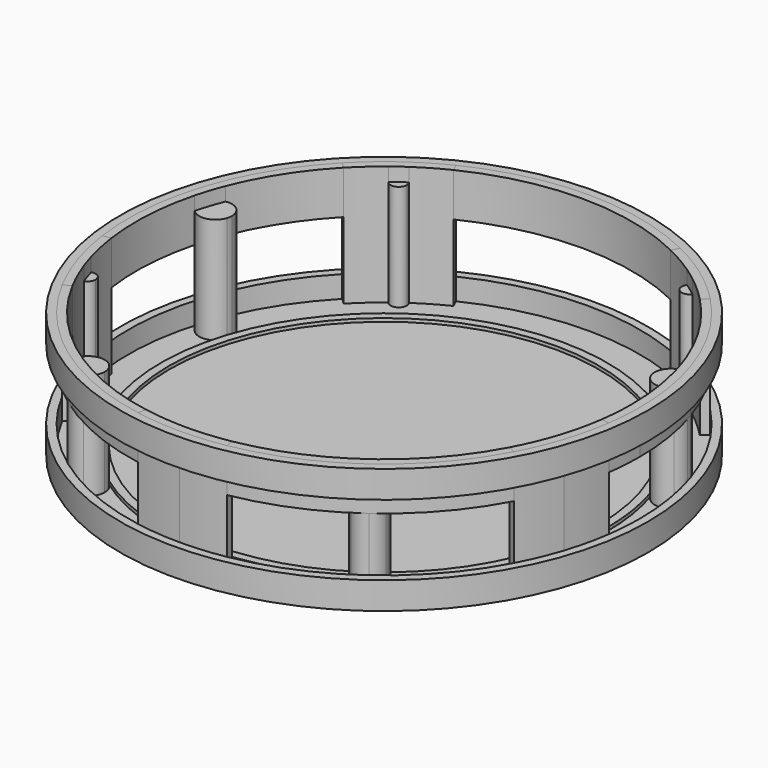
from build123d import *

# Parameters (mm, degrees)
F0_R     = 39.5
F1_DEPTH = 1
F2_DEPTH = 1.6
F3_DEPTH = 20.5
F4_DEPTH = 23
F5_START = 15
F5_DEPTH = 8
F0_R_2   = 48.5
F6_DEPTH = 5
F7_START = 18
F7_DEPTH = 5


with BuildPart() as f1:
    # F0 (on Top) → F1 (new body)
    with BuildSketch(Plane.XY):
        Circle(F0_R)
    extrude(amount=F1_DEPTH)


with BuildPart() as f1b:
    # F0 (on Top) → F1, piece 2 (new body)
    with BuildSketch(Plane.XY):
        with BuildLine():
            ThreePointArc((24.0991953374, -33.1696967742), (-9.68e-08, -41), (-24.099195494, -33.1696966604))
            ThreePointArc((-24.099195494, -33.1696966604), (-23.1895315704, -34.2347761707), (-22.8625511009, -35.5967477525))
            ThreePointArc((-22.8625511009, -35.5967477525), (-23.3228890862, -37.1936562819), (-24.5626290017, -38.3004863745))
            ThreePointArc((-24.5626290017, -38.3004863745), (-16.5547895287, -42.3814693429), (-7.9009920838, -44.8087527621))
            ThreePointArc((-7.9009920838, -44.8087527621), (-4.7121935446, -45.2553337409), (-1.4997962064, -45.4752747253))
            ThreePointArc((-1.4997962064, -45.4752747253), (0, -44), (1.4997962064, -45.4752747253))
            ThreePointArc((1.4997962064, -45.4752747253), (4.7121935446, -45.2553337409), (7.9009920838, -44.8087527621))
            ThreePointArc((7.9009920838, -44.8087527621), (16.5547895287, -42.3814693429), (24.5626290017, -38.3004863745))
            ThreePointArc((24.5626290017, -38.3004863745), (22.8747143756, -35.8666212476), (24.0991953374, -33.1696967742))
        make_face()
        with BuildLine():
            ThreePointArc((-24.5626290017, -38.3004863745), (-26.1324246507, -38.5845844728), (-27.6259069533, -38.0237986662))
            ThreePointArc((-27.6259069533, -38.0237986662), (-18.3643630933, -43.2637280892), (-8.1614643503, -46.2859643916))
            Line((-8.1614643503, -46.2859643916), (-7.9009920838, -44.8087527621))
            ThreePointArc((-7.9009920838, -44.8087527621), (-16.5547895287, -42.3814693429), (-24.5626290017, -38.3004863745))
        make_face()
        with BuildLine():
            ThreePointArc((8.1614643503, -46.2859643916), (18.3643629027, -43.2637281701), (27.6259066181, -38.0237989097))
            ThreePointArc((27.6259066181, -38.0237989097), (26.1324244444, -38.5845844914), (24.5626290017, -38.3004863745))
            ThreePointArc((24.5626290017, -38.3004863745), (16.5547895287, -42.3814693429), (7.9009920838, -44.8087527621))
            Line((7.9009920838, -44.8087527621), (8.1614643503, -46.2859643916))
        make_face()
    extrude(amount=F1_DEPTH)


with BuildPart() as f1c:
    # F0 (on Top) → F1, piece 3 (new body)
    with BuildSketch(Plane.XY):
        with BuildLine():
            ThreePointArc((45.5, 0), (45.1275246407, 5.8100361274), (44.0161969318, 11.5249471869))
            ThreePointArc((44.0161969318, 11.5249471869), (41.1798592989, 10.6717506781), (38.9933171455, 12.669696839))
            ThreePointArc((38.9933171455, 12.669696839), (40.4952219587, 6.4138131028), (41, 0))
            ThreePointArc((41, 0), (36.5312674899, -18.613610493), (24.0991953374, -33.1696967742))
            ThreePointArc((24.0991953374, -33.1696967742), (27.0425083639, -32.8385416584), (28.8356573557, -35.195949552))
            ThreePointArc((28.8356573557, -35.195949552), (35.191461286, -28.8411347307), (40.1741154751, -21.3609561068))
            ThreePointArc((40.1741154751, -21.3609561068), (41.5842321653, -18.4662295886), (42.7860938419, -15.4790236692))
            ThreePointArc((42.7860938419, -15.4790236692), (41.846486717, -13.5967477525), (43.7130188737, -12.6262417587))
            ThreePointArc((43.7130188737, -12.6262417587), (44.4965279374, -9.5031048354), (45.0571971277, -6.3323760937))
            ThreePointArc((45.0571971277, -6.3323760937), (45.3891642868, -3.1739195554), (45.5, 0))
        make_face()
        with BuildLine():
            ThreePointArc((27.6259066181, -38.0237989097), (35.4713501733, -30.8347744743), (41.4985368644, -22.0651634509))
            Line((41.4985368644, -22.0651634509), (40.1741154751, -21.3609561068))
            ThreePointArc((40.1741154751, -21.3609561068), (35.191461286, -28.8411347307), (28.8356573557, -35.195949552))
            ThreePointArc((28.8356573557, -35.195949552), (28.8558201135, -35.3958980132), (28.8625511009, -35.5967477525))
            ThreePointArc((28.8625511009, -35.5967477525), (28.5355706062, -36.9587193837), (27.6259066181, -38.0237989097))
        make_face()
        with BuildLine():
            ThreePointArc((47, 0), (46.4213520001, 7.3524199067), (44.6996562347, 14.5237988315))
            ThreePointArc((44.6996562347, 14.5237988315), (44.8095517309, 14.0660511974), (44.846486717, 13.5967477525))
            ThreePointArc((44.846486717, 13.5967477525), (44.6311887338, 12.4807573055), (44.0161969318, 11.5249471869))
            ThreePointArc((44.0161969318, 11.5249471869), (45.1275246407, 5.8100361274), (45.5, 0))
            ThreePointArc((45.5, 0), (45.3891642868, -3.1739195554), (45.0571971277, -6.3323760937))
            Line((45.0571971277, -6.3323760937), (46.5425992309, -6.5411357451))
            ThreePointArc((46.5425992309, -6.5411357451), (46.8855103622, -3.278554266), (47, 0))
        make_face()
    extrude(amount=F1_DEPTH)


with BuildPart() as f1d:
    # F0 (on Top) → F1, piece 4 (new body)
    with BuildSketch(Plane.XY):
        with BuildLine():
            ThreePointArc((25.5163352084, 37.6718281682), (22.7881731021, 39.3820919539), (19.9458871789, 40.8951291066))
            ThreePointArc((19.9458871789, 40.8951291066), (0, 45.5), (-19.9458871789, 40.8951291066))
            ThreePointArc((-19.9458871789, 40.8951291066), (-22.7881731021, 39.3820919539), (-25.5163352084, 37.6718281682))
            ThreePointArc((-25.5163352084, 37.6718281682), (-25.3138722657, 37.2620250252), (-25.2442289793, 36.8102732441))
            ThreePointArc((-25.2442289793, 36.8102732441), (-26.2689612657, 35.38755732), (-27.9430564466, 35.908711985))
            ThreePointArc((-27.9430564466, 35.908711985), (-30.4126624188, 33.842576211), (-32.7299609154, 31.6069558559))
            ThreePointArc((-32.7299609154, 31.6069558559), (-38.3043087172, 24.5566678052), (-42.3840453355, 16.5481932851))
            ThreePointArc((-42.3840453355, 16.5481932851), (-39.9245964828, 15.9002967378), (-38.846486717, 13.5967477525))
            ThreePointArc((-38.846486717, 13.5967477525), (-38.8834216837, 13.12744443), (-38.9933171226, 12.6696969093))
            ThreePointArc((-38.9933171226, 12.6696969093), (3.7e-08, 41), (38.9933171455, 12.669696839))
            ThreePointArc((38.9933171455, 12.669696839), (39.5879037117, 15.5712863842), (42.3840453355, 16.5481932851))
            ThreePointArc((42.3840453355, 16.5481932851), (38.3043087172, 24.5566678052), (32.7299609154, 31.6069558559))
            ThreePointArc((32.7299609154, 31.6069558559), (30.4126624188, 33.842576211), (27.9430564466, 35.908711985))
            ThreePointArc((27.9430564466, 35.908711985), (25.8625511009, 35.5967477525), (25.5163352084, 37.6718281682))
        make_face()
        with BuildLine():
            ThreePointArc((44.6996562347, 14.5237988315), (40.286863107, 24.206789564), (33.8089706159, 32.6489434116))
            Line((33.8089706159, 32.6489434116), (32.7299609154, 31.6069558559))
            ThreePointArc((32.7299609154, 31.6069558559), (38.3043087172, 24.5566678052), (42.3840453355, 16.5481932851))
            ThreePointArc((42.3840453355, 16.5481932851), (43.8210252832, 15.8553308151), (44.6996562347, 14.5237988315))
        make_face()
        with BuildLine():
            Line((19.9458871789, 40.8951291066), (20.6034438991, 42.2433201761))
            ThreePointArc((20.6034438991, 42.2433201761), (0, 47), (-20.6034438991, 42.2433201761))
            Line((-20.6034438991, 42.2433201761), (-19.9458871789, 40.8951291066))
            ThreePointArc((-19.9458871789, 40.8951291066), (0, 45.5), (19.9458871789, 40.8951291066))
        make_face()
        with BuildLine():
            Line((-32.7299609154, 31.6069558559), (-33.8089706159, 32.6489434116))
            ThreePointArc((-33.8089706159, 32.6489434116), (-40.2868630773, 24.2067896134), (-44.6996561991, 14.5237989412))
            ThreePointArc((-44.6996561991, 14.5237989412), (-43.8210252397, 15.8553308531), (-42.3840453355, 16.5481932851))
            ThreePointArc((-42.3840453355, 16.5481932851), (-38.3043087172, 24.5566678052), (-32.7299609154, 31.6069558559))
        make_face()
    extrude(amount=F1_DEPTH)


with BuildPart() as f1e:
    # F0 (on Top) → F1, piece 5 (new body)
    with BuildSketch(Plane.XY):
        with BuildLine():
            ThreePointArc((-38.9933171226, 12.6696969093), (-41.1798592628, 10.6717506863), (-44.0161969318, 11.5249471869))
            ThreePointArc((-44.0161969318, 11.5249471869), (-45.4228838914, 2.6479461836), (-45.0571971277, -6.3323760937))
            ThreePointArc((-45.0571971277, -6.3323760937), (-44.4965279374, -9.5031048354), (-43.7130188737, -12.6262417587))
            ThreePointArc((-43.7130188737, -12.6262417587), (-42.3814216368, -12.8540557941), (-41.7730714914, -14.0602732441))
            ThreePointArc((-41.7730714914, -14.0602732441), (-42.0523203959, -14.9319192518), (-42.7860938419, -15.4790236692))
            ThreePointArc((-42.7860938419, -15.4790236692), (-41.5842321653, -18.4662295886), (-40.1741154751, -21.3609561068))
            ThreePointArc((-40.1741154751, -21.3609561068), (-35.191461286, -28.8411347307), (-28.8356573557, -35.195949552))
            ThreePointArc((-28.8356573557, -35.195949552), (-27.0425084529, -32.8385416965), (-24.099195494, -33.1696966604))
            ThreePointArc((-24.099195494, -33.1696966604), (-38.9933172195, -12.6696966113), (-38.9933171226, 12.6696969093))
        make_face()
        with BuildLine():
            Line((-40.1741154751, -21.3609561068), (-41.4985368644, -22.0651634509))
            ThreePointArc((-41.4985368644, -22.0651634509), (-35.4713503092, -30.834774318), (-27.6259069533, -38.0237986662))
            ThreePointArc((-27.6259069533, -38.0237986662), (-28.6207572165, -36.7767049651), (-28.8356573557, -35.195949552))
            ThreePointArc((-28.8356573557, -35.195949552), (-35.191461286, -28.8411347307), (-40.1741154751, -21.3609561068))
        make_face()
        with BuildLine():
            ThreePointArc((-44.0161969318, 11.5249471869), (-44.7714838236, 12.9301204755), (-44.6996561991, 14.5237989412))
            ThreePointArc((-44.6996561991, 14.5237989412), (-46.8211508009, 4.0963200168), (-46.5425992309, -6.5411357451))
            Line((-46.5425992309, -6.5411357451), (-45.0571971277, -6.3323760937))
            ThreePointArc((-45.0571971277, -6.3323760937), (-45.4228838914, 2.6479461836), (-44.0161969318, 11.5249471869))
        make_face()
    extrude(amount=F1_DEPTH)


with BuildPart() as f2:
    # F0 (on Top) → F2 (new body)
    with BuildSketch(Plane.XY):
        with BuildLine():
            ThreePointArc((41, 0), (40.4952219587, 6.4138131028), (38.9933171455, 12.669696839))
            ThreePointArc((38.9933171455, 12.669696839), (3.7e-08, 41), (-38.9933171226, 12.6696969093))
            ThreePointArc((-38.9933171226, 12.6696969093), (-38.9933172195, -12.6696966113), (-24.099195494, -33.1696966604))
            ThreePointArc((-24.099195494, -33.1696966604), (-9.68e-08, -41), (24.0991953374, -33.1696967742))
            ThreePointArc((24.0991953374, -33.1696967742), (36.5312674899, -18.613610493), (41, 0))
        make_face()
        Circle(F0_R, mode=Mode.SUBTRACT)
    extrude(amount=F2_DEPTH)


with BuildPart() as f3:
    # F0 (on Top) → F3 (new body)
    with BuildSketch(Plane.XY):
        with BuildLine():
            ThreePointArc((27.9430564466, 35.908711985), (26.7442289793, 36.8102732441), (25.5163352084, 37.6718281682))
            ThreePointArc((25.5163352084, 37.6718281682), (25.8625511009, 35.5967477525), (27.9430564466, 35.908711985))
        make_face()
    extrude(amount=F3_DEPTH)


with BuildPart() as f3b:
    # F0 (on Top) → F3, piece 2 (new body)
    with BuildSketch(Plane.XY):
        with BuildLine():
            ThreePointArc((-25.2442289793, 36.8102732441), (-25.3138722657, 37.2620250252), (-25.5163352084, 37.6718281682))
            ThreePointArc((-25.5163352084, 37.6718281682), (-26.7442289793, 36.8102732441), (-27.9430564466, 35.908711985))
            ThreePointArc((-27.9430564466, 35.908711985), (-26.2689612657, 35.38755732), (-25.2442289793, 36.8102732441))
        make_face()
    extrude(amount=F3_DEPTH)


with BuildPart() as f3c:
    # F0 (on Top) → F3, piece 3 (new body)
    with BuildSketch(Plane.XY):
        with BuildLine():
            ThreePointArc((44.846486717, 13.5967477525), (44.8095517309, 14.0660511974), (44.6996562347, 14.5237988315))
            ThreePointArc((44.6996562347, 14.5237988315), (43.8210252832, 15.8553308151), (42.3840453355, 16.5481932851))
            ThreePointArc((42.3840453355, 16.5481932851), (43.2730714914, 14.0602732441), (44.0161969318, 11.5249471869))
            ThreePointArc((44.0161969318, 11.5249471869), (44.6311887338, 12.4807573055), (44.846486717, 13.5967477525))
        make_face()
        with BuildLine():
            ThreePointArc((44.0161969318, 11.5249471869), (43.2730714914, 14.0602732441), (42.3840453355, 16.5481932851))
            ThreePointArc((42.3840453355, 16.5481932851), (39.5879037117, 15.5712863842), (38.9933171455, 12.669696839))
            ThreePointArc((38.9933171455, 12.669696839), (41.1798592989, 10.6717506781), (44.0161969318, 11.5249471869))
        make_face()
    extrude(amount=F3_DEPTH)


with BuildPart() as f3d:
    # F0 (on Top) → F3, piece 4 (new body)
    with BuildSketch(Plane.XY):
        with BuildLine():
            ThreePointArc((-42.3840453355, 16.5481932851), (-43.8210252397, 15.8553308531), (-44.6996561991, 14.5237989412))
            ThreePointArc((-44.6996561991, 14.5237989412), (-44.7714838236, 12.9301204755), (-44.0161969318, 11.5249471869))
            ThreePointArc((-44.0161969318, 11.5249471869), (-43.2730714914, 14.0602732441), (-42.3840453355, 16.5481932851))
        make_face()
        with BuildLine():
            ThreePointArc((-38.846486717, 13.5967477525), (-39.9245964828, 15.9002967378), (-42.3840453355, 16.5481932851))
            ThreePointArc((-42.3840453355, 16.5481932851), (-43.2730714914, 14.0602732441), (-44.0161969318, 11.5249471869))
            ThreePointArc((-44.0161969318, 11.5249471869), (-41.1798592628, 10.6717506863), (-38.9933171226, 12.6696969093))
            ThreePointArc((-38.9933171226, 12.6696969093), (-38.8834216837, 13.12744443), (-38.846486717, 13.5967477525))
        make_face()
    extrude(amount=F3_DEPTH)


with BuildPart() as f3e:
    # F0 (on Top) → F3, piece 5 (new body)
    with BuildSketch(Plane.XY):
        with BuildLine():
            ThreePointArc((-41.7730714914, -14.0602732441), (-42.3814216368, -12.8540557941), (-43.7130188737, -12.6262417587))
            ThreePointArc((-43.7130188737, -12.6262417587), (-43.2730714914, -14.0602732441), (-42.7860938419, -15.4790236692))
            ThreePointArc((-42.7860938419, -15.4790236692), (-42.0523203959, -14.9319192518), (-41.7730714914, -14.0602732441))
        make_face()
    extrude(amount=F3_DEPTH)


with BuildPart() as f3f:
    # F0 (on Top) → F3, piece 6 (new body)
    with BuildSketch(Plane.XY):
        with BuildLine():
            ThreePointArc((-22.8625511009, -35.5967477525), (-23.1895315704, -34.2347761707), (-24.099195494, -33.1696966604))
            ThreePointArc((-24.099195494, -33.1696966604), (-27.0425084529, -32.8385416965), (-28.8356573557, -35.195949552))
            ThreePointArc((-28.8356573557, -35.195949552), (-26.7442289793, -36.8102732441), (-24.5626290017, -38.3004863745))
            ThreePointArc((-24.5626290017, -38.3004863745), (-23.3228890862, -37.1936562819), (-22.8625511009, -35.5967477525))
        make_face()
        with BuildLine():
            ThreePointArc((-28.8356573557, -35.195949552), (-28.6207572165, -36.7767049651), (-27.6259069533, -38.0237986662))
            ThreePointArc((-27.6259069533, -38.0237986662), (-26.1324246507, -38.5845844728), (-24.5626290017, -38.3004863745))
            ThreePointArc((-24.5626290017, -38.3004863745), (-26.7442289793, -36.8102732441), (-28.8356573557, -35.195949552))
        make_face()
    extrude(amount=F3_DEPTH)


with BuildPart() as f3g:
    # F0 (on Top) → F3, piece 7 (new body)
    with BuildSketch(Plane.XY):
        with BuildLine():
            ThreePointArc((43.7130188737, -12.6262417587), (41.846486717, -13.5967477525), (42.7860938419, -15.4790236692))
            ThreePointArc((42.7860938419, -15.4790236692), (43.2730714914, -14.0602732441), (43.7130188737, -12.6262417587))
        make_face()
    extrude(amount=F3_DEPTH)


with BuildPart() as f3h:
    # F0 (on Top) → F3, piece 8 (new body)
    with BuildSketch(Plane.XY):
        with BuildLine():
            ThreePointArc((28.8356573557, -35.195949552), (27.0425083639, -32.8385416584), (24.0991953374, -33.1696967742))
            ThreePointArc((24.0991953374, -33.1696967742), (22.8747143756, -35.8666212476), (24.5626290017, -38.3004863745))
            ThreePointArc((24.5626290017, -38.3004863745), (26.7442289793, -36.8102732441), (28.8356573557, -35.195949552))
        make_face()
        with BuildLine():
            ThreePointArc((24.5626290017, -38.3004863745), (26.1324244444, -38.5845844914), (27.6259066181, -38.0237989097))
            ThreePointArc((27.6259066181, -38.0237989097), (28.5355706062, -36.9587193837), (28.8625511009, -35.5967477525))
            ThreePointArc((28.8625511009, -35.5967477525), (28.8558201135, -35.3958980132), (28.8356573557, -35.195949552))
            ThreePointArc((28.8356573557, -35.195949552), (26.7442289793, -36.8102732441), (24.5626290017, -38.3004863745))
        make_face()
    extrude(amount=F3_DEPTH)


with BuildPart() as f3i:
    # F0 (on Top) → F3, piece 9 (new body)
    with BuildSketch(Plane.XY):
        with BuildLine():
            ThreePointArc((0, -45.5), (0.75, -45.4938182614), (1.4997962064, -45.4752747253))
            ThreePointArc((1.4997962064, -45.4752747253), (0, -44), (-1.4997962064, -45.4752747253))
            ThreePointArc((-1.4997962064, -45.4752747253), (-0.75, -45.4938182614), (0, -45.5))
        make_face()
    extrude(amount=F3_DEPTH)


with BuildPart() as f4:
    # F0 (on Top) → F4 (new body)
    with BuildSketch(Plane.XY):
        with BuildLine():
            ThreePointArc((-42.7860938419, -15.4790236692), (-43.9430185539, -15.4023503408), (-44.6996562714, -14.5237987185))
            ThreePointArc((-44.6996562714, -14.5237987185), (-43.2637281158, -18.3643630307), (-41.4985368644, -22.0651634509))
            Line((-41.4985368644, -22.0651634509), (-40.1741154751, -21.3609561068))
            ThreePointArc((-40.1741154751, -21.3609561068), (-41.5842321653, -18.4662295886), (-42.7860938419, -15.4790236692))
        make_face()
        with BuildLine():
            ThreePointArc((-43.7130188737, -12.6262417587), (-44.6039231669, -13.3682950523), (-44.6996562714, -14.5237987185))
            ThreePointArc((-44.6996562714, -14.5237987185), (-43.9430185539, -15.4023503408), (-42.7860938419, -15.4790236692))
            ThreePointArc((-42.7860938419, -15.4790236692), (-43.2730714914, -14.0602732441), (-43.7130188737, -12.6262417587))
        make_face()
        with BuildLine():
            Line((-45.0571971277, -6.3323760937), (-46.5425992309, -6.5411357451))
            ThreePointArc((-46.5425992309, -6.5411357451), (-45.7953930469, -10.5726995454), (-44.6996562714, -14.5237987185))
            ThreePointArc((-44.6996562714, -14.5237987185), (-44.6039231669, -13.3682950523), (-43.7130188737, -12.6262417587))
            ThreePointArc((-43.7130188737, -12.6262417587), (-44.4965279374, -9.5031048354), (-45.0571971277, -6.3323760937))
        make_face()
    extrude(amount=F4_DEPTH)


with BuildPart() as f4b:
    # F0 (on Top) → F4, piece 2 (new body)
    with BuildSketch(Plane.XY):
        with BuildLine():
            ThreePointArc((-27.9430564466, 35.908711985), (-28.2276451659, 37.0327061945), (-27.6259067422, 38.0237988196))
            ThreePointArc((-27.6259067422, 38.0237988196), (-30.8347743086, 35.4713503173), (-33.8089706159, 32.6489434116))
            Line((-33.8089706159, 32.6489434116), (-32.7299609154, 31.6069558559))
            ThreePointArc((-32.7299609154, 31.6069558559), (-30.4126624188, 33.842576211), (-27.9430564466, 35.908711985))
        make_face()
        with BuildLine():
            ThreePointArc((-25.5163352084, 37.6718281682), (-26.497374334, 38.289821413), (-27.6259067422, 38.0237988196))
            ThreePointArc((-27.6259067422, 38.0237988196), (-28.2276451659, 37.0327061945), (-27.9430564466, 35.908711985))
            ThreePointArc((-27.9430564466, 35.908711985), (-26.7442289793, 36.8102732441), (-25.5163352084, 37.6718281682))
        make_face()
        with BuildLine():
            Line((-19.9458871789, 40.8951291066), (-20.6034438991, 42.2433201761))
            ThreePointArc((-20.6034438991, 42.2433201761), (-24.2067894595, 40.2868631698), (-27.6259067422, 38.0237988196))
            ThreePointArc((-27.6259067422, 38.0237988196), (-26.497374334, 38.289821413), (-25.5163352084, 37.6718281682))
            ThreePointArc((-25.5163352084, 37.6718281682), (-22.7881731021, 39.3820919539), (-19.9458871789, 40.8951291066))
        make_face()
    extrude(amount=F4_DEPTH)


with BuildPart() as f4c:
    # F0 (on Top) → F4, piece 3 (new body)
    with BuildSketch(Plane.XY):
        with BuildLine():
            ThreePointArc((28.2442289793, 36.8102732441), (28.0807387591, 37.4912590064), (27.6259068347, 38.0237987524))
            ThreePointArc((27.6259068347, 38.0237987524), (26.4973743904, 38.2898214224), (25.5163352084, 37.6718281682))
            ThreePointArc((25.5163352084, 37.6718281682), (26.7442289793, 36.8102732441), (27.9430564466, 35.908711985))
            ThreePointArc((27.9430564466, 35.908711985), (28.1669449033, 36.3350055305), (28.2442289793, 36.8102732441))
        make_face()
        with BuildLine():
            ThreePointArc((27.6259068347, 38.0237987524), (24.2067895086, 40.2868631403), (20.6034438991, 42.2433201761))
            Line((20.6034438991, 42.2433201761), (19.9458871789, 40.8951291066))
            ThreePointArc((19.9458871789, 40.8951291066), (22.7881731021, 39.3820919539), (25.5163352084, 37.6718281682))
            ThreePointArc((25.5163352084, 37.6718281682), (26.4973743904, 38.2898214224), (27.6259068347, 38.0237987524))
        make_face()
        with BuildLine():
            ThreePointArc((33.8089706159, 32.6489434116), (30.8347743518, 35.4713502798), (27.6259068347, 38.0237987524))
            ThreePointArc((27.6259068347, 38.0237987524), (28.0807387591, 37.4912590064), (28.2442289793, 36.8102732441))
            ThreePointArc((28.2442289793, 36.8102732441), (28.1669449033, 36.3350055305), (27.9430564466, 35.908711985))
            ThreePointArc((27.9430564466, 35.908711985), (30.4126624188, 33.842576211), (32.7299609154, 31.6069558559))
            Line((32.7299609154, 31.6069558559), (33.8089706159, 32.6489434116))
        make_face()
    extrude(amount=F4_DEPTH)


with BuildPart() as f4d:
    # F0 (on Top) → F4, piece 4 (new body)
    with BuildSketch(Plane.XY):
        with BuildLine():
            ThreePointArc((42.7860938419, -15.4790236692), (43.9430184652, -15.402350385), (44.6996562102, -14.523798907))
            ThreePointArc((44.6996562102, -14.523798907), (44.7546039882, -14.2949250306), (44.7730714914, -14.0602732441))
            ThreePointArc((44.7730714914, -14.0602732441), (44.4792889414, -13.1686233894), (43.7130188737, -12.6262417587))
            ThreePointArc((43.7130188737, -12.6262417587), (43.2730714914, -14.0602732441), (42.7860938419, -15.4790236692))
        make_face()
        with BuildLine():
            ThreePointArc((44.6996562102, -14.523798907), (45.7953930246, -10.572699642), (46.5425992309, -6.5411357451))
            Line((46.5425992309, -6.5411357451), (45.0571971277, -6.3323760937))
            ThreePointArc((45.0571971277, -6.3323760937), (44.4965279374, -9.5031048354), (43.7130188737, -12.6262417587))
            ThreePointArc((43.7130188737, -12.6262417587), (44.4792889414, -13.1686233894), (44.7730714914, -14.0602732441))
            ThreePointArc((44.7730714914, -14.0602732441), (44.7546039882, -14.2949250306), (44.6996562102, -14.523798907))
        make_face()
        with BuildLine():
            ThreePointArc((41.4985368644, -22.0651634509), (43.2637280771, -18.3643631219), (44.6996562102, -14.523798907))
            ThreePointArc((44.6996562102, -14.523798907), (43.9430184652, -15.402350385), (42.7860938419, -15.4790236692))
            ThreePointArc((42.7860938419, -15.4790236692), (41.5842321653, -18.4662295886), (40.1741154751, -21.3609561068))
            Line((40.1741154751, -21.3609561068), (41.4985368644, -22.0651634509))
        make_face()
    extrude(amount=F4_DEPTH)


with BuildPart() as f4e:
    # F0 (on Top) → F4, piece 5 (new body)
    with BuildSketch(Plane.XY):
        with BuildLine():
            ThreePointArc((-1.4997962064, -45.4752747253), (-1.0693661469, -46.5518821436), (0, -47))
            Line((0, -47), (0, -45.5))
            ThreePointArc((0, -45.5), (-0.75, -45.4938182614), (-1.4997962064, -45.4752747253))
        make_face()
        with BuildLine():
            Line((0, -45.5), (0, -47))
            ThreePointArc((0, -47), (1.0606601718, -46.5606601718), (1.5, -45.5))
            ThreePointArc((1.5, -45.5), (1.4999490507, -45.4876369427), (1.4997962064, -45.4752747253))
            ThreePointArc((1.4997962064, -45.4752747253), (0.75, -45.4938182614), (0, -45.5))
        make_face()
        with BuildLine():
            ThreePointArc((0, -47), (4.0963199091, -46.8211508103), (8.1614643503, -46.2859643916))
            Line((8.1614643503, -46.2859643916), (7.9009920838, -44.8087527621))
            ThreePointArc((7.9009920838, -44.8087527621), (4.7121935446, -45.2553337409), (1.4997962064, -45.4752747253))
            ThreePointArc((1.4997962064, -45.4752747253), (1.4999490507, -45.4876369427), (1.5, -45.5))
            ThreePointArc((1.5, -45.5), (1.0606601718, -46.5606601718), (0, -47))
        make_face()
        with BuildLine():
            Line((-7.9009920838, -44.8087527621), (-8.1614643503, -46.2859643916))
            ThreePointArc((-8.1614643503, -46.2859643916), (-4.0963199091, -46.8211508103), (0, -47))
            ThreePointArc((0, -47), (-1.0693661469, -46.5518821436), (-1.4997962064, -45.4752747253))
            ThreePointArc((-1.4997962064, -45.4752747253), (-4.7121935446, -45.2553337409), (-7.9009920838, -44.8087527621))
        make_face()
    extrude(amount=F4_DEPTH)


with BuildPart() as f5:
    # F0 (on Top) → F5 (new body)
    with BuildSketch(Plane.XY.offset(F5_START)):
        with BuildLine():
            ThreePointArc((-42.3840453355, 16.5481932851), (-43.8210252397, 15.8553308531), (-44.6996561991, 14.5237989412))
            ThreePointArc((-44.6996561991, 14.5237989412), (-44.7714838236, 12.9301204755), (-44.0161969318, 11.5249471869))
            ThreePointArc((-44.0161969318, 11.5249471869), (-43.2730714914, 14.0602732441), (-42.3840453355, 16.5481932851))
        make_face()
        with BuildLine():
            Line((-32.7299609154, 31.6069558559), (-33.8089706159, 32.6489434116))
            ThreePointArc((-33.8089706159, 32.6489434116), (-40.2868630773, 24.2067896134), (-44.6996561991, 14.5237989412))
            ThreePointArc((-44.6996561991, 14.5237989412), (-43.8210252397, 15.8553308531), (-42.3840453355, 16.5481932851))
            ThreePointArc((-42.3840453355, 16.5481932851), (-38.3043087172, 24.5566678052), (-32.7299609154, 31.6069558559))
        make_face()
        with BuildLine():
            ThreePointArc((-44.0161969318, 11.5249471869), (-44.7714838236, 12.9301204755), (-44.6996561991, 14.5237989412))
            ThreePointArc((-44.6996561991, 14.5237989412), (-46.8211508009, 4.0963200168), (-46.5425992309, -6.5411357451))
            Line((-46.5425992309, -6.5411357451), (-45.0571971277, -6.3323760937))
            ThreePointArc((-45.0571971277, -6.3323760937), (-45.4228838914, 2.6479461836), (-44.0161969318, 11.5249471869))
        make_face()
    extrude(amount=F5_DEPTH)


with BuildPart() as f5b:
    # F0 (on Top) → F5, piece 2 (new body)
    with BuildSketch(Plane.XY.offset(F5_START)):
        with BuildLine():
            ThreePointArc((-28.8356573557, -35.195949552), (-28.6207572165, -36.7767049651), (-27.6259069533, -38.0237986662))
            ThreePointArc((-27.6259069533, -38.0237986662), (-26.1324246507, -38.5845844728), (-24.5626290017, -38.3004863745))
            ThreePointArc((-24.5626290017, -38.3004863745), (-26.7442289793, -36.8102732441), (-28.8356573557, -35.195949552))
        make_face()
        with BuildLine():
            Line((-40.1741154751, -21.3609561068), (-41.4985368644, -22.0651634509))
            ThreePointArc((-41.4985368644, -22.0651634509), (-35.4713503092, -30.834774318), (-27.6259069533, -38.0237986662))
            ThreePointArc((-27.6259069533, -38.0237986662), (-28.6207572165, -36.7767049651), (-28.8356573557, -35.195949552))
            ThreePointArc((-28.8356573557, -35.195949552), (-35.191461286, -28.8411347307), (-40.1741154751, -21.3609561068))
        make_face()
        with BuildLine():
            ThreePointArc((-24.5626290017, -38.3004863745), (-26.1324246507, -38.5845844728), (-27.6259069533, -38.0237986662))
            ThreePointArc((-27.6259069533, -38.0237986662), (-18.3643630933, -43.2637280892), (-8.1614643503, -46.2859643916))
            Line((-8.1614643503, -46.2859643916), (-7.9009920838, -44.8087527621))
            ThreePointArc((-7.9009920838, -44.8087527621), (-16.5547895287, -42.3814693429), (-24.5626290017, -38.3004863745))
        make_face()
    extrude(amount=F5_DEPTH)


with BuildPart() as f5c:
    # F0 (on Top) → F5, piece 3 (new body)
    with BuildSketch(Plane.XY.offset(F5_START)):
        with BuildLine():
            ThreePointArc((24.5626290017, -38.3004863745), (26.1324244444, -38.5845844914), (27.6259066181, -38.0237989097))
            ThreePointArc((27.6259066181, -38.0237989097), (28.5355706062, -36.9587193837), (28.8625511009, -35.5967477525))
            ThreePointArc((28.8625511009, -35.5967477525), (28.8558201135, -35.3958980132), (28.8356573557, -35.195949552))
            ThreePointArc((28.8356573557, -35.195949552), (26.7442289793, -36.8102732441), (24.5626290017, -38.3004863745))
        make_face()
        with BuildLine():
            ThreePointArc((27.6259066181, -38.0237989097), (35.4713501733, -30.8347744743), (41.4985368644, -22.0651634509))
            Line((41.4985368644, -22.0651634509), (40.1741154751, -21.3609561068))
            ThreePointArc((40.1741154751, -21.3609561068), (35.191461286, -28.8411347307), (28.8356573557, -35.195949552))
            ThreePointArc((28.8356573557, -35.195949552), (28.8558201135, -35.3958980132), (28.8625511009, -35.5967477525))
            ThreePointArc((28.8625511009, -35.5967477525), (28.5355706062, -36.9587193837), (27.6259066181, -38.0237989097))
        make_face()
        with BuildLine():
            ThreePointArc((8.1614643503, -46.2859643916), (18.3643629027, -43.2637281701), (27.6259066181, -38.0237989097))
            ThreePointArc((27.6259066181, -38.0237989097), (26.1324244444, -38.5845844914), (24.5626290017, -38.3004863745))
            ThreePointArc((24.5626290017, -38.3004863745), (16.5547895287, -42.3814693429), (7.9009920838, -44.8087527621))
            Line((7.9009920838, -44.8087527621), (8.1614643503, -46.2859643916))
        make_face()
    extrude(amount=F5_DEPTH)


with BuildPart() as f5d:
    # F0 (on Top) → F5, piece 4 (new body)
    with BuildSketch(Plane.XY.offset(F5_START)):
        with BuildLine():
            ThreePointArc((44.846486717, 13.5967477525), (44.8095517309, 14.0660511974), (44.6996562347, 14.5237988315))
            ThreePointArc((44.6996562347, 14.5237988315), (43.8210252832, 15.8553308151), (42.3840453355, 16.5481932851))
            ThreePointArc((42.3840453355, 16.5481932851), (43.2730714914, 14.0602732441), (44.0161969318, 11.5249471869))
            ThreePointArc((44.0161969318, 11.5249471869), (44.6311887338, 12.4807573055), (44.846486717, 13.5967477525))
        make_face()
        with BuildLine():
            ThreePointArc((44.6996562347, 14.5237988315), (40.286863107, 24.206789564), (33.8089706159, 32.6489434116))
            Line((33.8089706159, 32.6489434116), (32.7299609154, 31.6069558559))
            ThreePointArc((32.7299609154, 31.6069558559), (38.3043087172, 24.5566678052), (42.3840453355, 16.5481932851))
            ThreePointArc((42.3840453355, 16.5481932851), (43.8210252832, 15.8553308151), (44.6996562347, 14.5237988315))
        make_face()
        with BuildLine():
            ThreePointArc((47, 0), (46.4213520001, 7.3524199067), (44.6996562347, 14.5237988315))
            ThreePointArc((44.6996562347, 14.5237988315), (44.8095517309, 14.0660511974), (44.846486717, 13.5967477525))
            ThreePointArc((44.846486717, 13.5967477525), (44.6311887338, 12.4807573055), (44.0161969318, 11.5249471869))
            ThreePointArc((44.0161969318, 11.5249471869), (45.1275246407, 5.8100361274), (45.5, 0))
            ThreePointArc((45.5, 0), (45.3891642868, -3.1739195554), (45.0571971277, -6.3323760937))
            Line((45.0571971277, -6.3323760937), (46.5425992309, -6.5411357451))
            ThreePointArc((46.5425992309, -6.5411357451), (46.8855103622, -3.278554266), (47, 0))
        make_face()
    extrude(amount=F5_DEPTH)


with BuildPart() as f5e:
    # F0 (on Top) → F5, piece 5 (new body)
    with BuildSketch(Plane.XY.offset(F5_START)):
        with BuildLine():
            Line((19.9458871789, 40.8951291066), (20.6034438991, 42.2433201761))
            ThreePointArc((20.6034438991, 42.2433201761), (0, 47), (-20.6034438991, 42.2433201761))
            Line((-20.6034438991, 42.2433201761), (-19.9458871789, 40.8951291066))
            ThreePointArc((-19.9458871789, 40.8951291066), (0, 45.5), (19.9458871789, 40.8951291066))
        make_face()
    extrude(amount=F5_DEPTH)


with BuildPart() as f6:
    # F0 (on Top) → F6 (new body)
    with BuildSketch(Plane.XY):
        Circle(F0_R_2)
        with BuildLine():
            ThreePointArc((-20.6034438991, 42.2433201761), (0, 47), (20.6034438991, 42.2433201761))
            ThreePointArc((20.6034438991, 42.2433201761), (24.2067895086, 40.2868631403), (27.6259068347, 38.0237987524))
            ThreePointArc((27.6259068347, 38.0237987524), (30.8347743518, 35.4713502798), (33.8089706159, 32.6489434116))
            ThreePointArc((33.8089706159, 32.6489434116), (40.286863107, 24.206789564), (44.6996562347, 14.5237988315))
            ThreePointArc((44.6996562347, 14.5237988315), (46.4213520001, 7.3524199067), (47, 0))
            ThreePointArc((47, 0), (46.8855103622, -3.278554266), (46.5425992309, -6.5411357451))
            ThreePointArc((46.5425992309, -6.5411357451), (45.7953930246, -10.572699642), (44.6996562102, -14.523798907))
            ThreePointArc((44.6996562102, -14.523798907), (43.2637280771, -18.3643631219), (41.4985368644, -22.0651634509))
            ThreePointArc((41.4985368644, -22.0651634509), (35.4713501733, -30.8347744743), (27.6259066181, -38.0237989097))
            ThreePointArc((27.6259066181, -38.0237989097), (18.3643629027, -43.2637281701), (8.1614643503, -46.2859643916))
            ThreePointArc((8.1614643503, -46.2859643916), (4.0963199091, -46.8211508103), (0, -47))
            ThreePointArc((0, -47), (-4.0963199091, -46.8211508103), (-8.1614643503, -46.2859643916))
            ThreePointArc((-8.1614643503, -46.2859643916), (-18.3643630933, -43.2637280892), (-27.6259069533, -38.0237986662))
            ThreePointArc((-27.6259069533, -38.0237986662), (-35.4713503092, -30.834774318), (-41.4985368644, -22.0651634509))
            ThreePointArc((-41.4985368644, -22.0651634509), (-43.2637281158, -18.3643630307), (-44.6996562714, -14.5237987185))
            ThreePointArc((-44.6996562714, -14.5237987185), (-45.7953930469, -10.5726995454), (-46.5425992309, -6.5411357451))
            ThreePointArc((-46.5425992309, -6.5411357451), (-46.8211508009, 4.0963200168), (-44.6996561991, 14.5237989412))
            ThreePointArc((-44.6996561991, 14.5237989412), (-40.2868630773, 24.2067896134), (-33.8089706159, 32.6489434116))
            ThreePointArc((-33.8089706159, 32.6489434116), (-30.8347743086, 35.4713503173), (-27.6259067422, 38.0237988196))
            ThreePointArc((-27.6259067422, 38.0237988196), (-24.2067894595, 40.2868631698), (-20.6034438991, 42.2433201761))
        make_face(mode=Mode.SUBTRACT)
    extrude(amount=F6_DEPTH)


with BuildPart() as f7:
    # F0 (on Top) → F7 (new body)
    with BuildSketch(Plane.XY.offset(F7_START)):
        Circle(F0_R_2)
        with BuildLine():
            ThreePointArc((-20.6034438991, 42.2433201761), (0, 47), (20.6034438991, 42.2433201761))
            ThreePointArc((20.6034438991, 42.2433201761), (24.2067895086, 40.2868631403), (27.6259068347, 38.0237987524))
            ThreePointArc((27.6259068347, 38.0237987524), (30.8347743518, 35.4713502798), (33.8089706159, 32.6489434116))
            ThreePointArc((33.8089706159, 32.6489434116), (40.286863107, 24.206789564), (44.6996562347, 14.5237988315))
            ThreePointArc((44.6996562347, 14.5237988315), (46.4213520001, 7.3524199067), (47, 0))
            ThreePointArc((47, 0), (46.8855103622, -3.278554266), (46.5425992309, -6.5411357451))
            ThreePointArc((46.5425992309, -6.5411357451), (45.7953930246, -10.572699642), (44.6996562102, -14.523798907))
            ThreePointArc((44.6996562102, -14.523798907), (43.2637280771, -18.3643631219), (41.4985368644, -22.0651634509))
            ThreePointArc((41.4985368644, -22.0651634509), (35.4713501733, -30.8347744743), (27.6259066181, -38.0237989097))
            ThreePointArc((27.6259066181, -38.0237989097), (18.3643629027, -43.2637281701), (8.1614643503, -46.2859643916))
            ThreePointArc((8.1614643503, -46.2859643916), (4.0963199091, -46.8211508103), (0, -47))
            ThreePointArc((0, -47), (-4.0963199091, -46.8211508103), (-8.1614643503, -46.2859643916))
            ThreePointArc((-8.1614643503, -46.2859643916), (-18.3643630933, -43.2637280892), (-27.6259069533, -38.0237986662))
            ThreePointArc((-27.6259069533, -38.0237986662), (-35.4713503092, -30.834774318), (-41.4985368644, -22.0651634509))
            ThreePointArc((-41.4985368644, -22.0651634509), (-43.2637281158, -18.3643630307), (-44.6996562714, -14.5237987185))
            ThreePointArc((-44.6996562714, -14.5237987185), (-45.7953930469, -10.5726995454), (-46.5425992309, -6.5411357451))
            ThreePointArc((-46.5425992309, -6.5411357451), (-46.8211508009, 4.0963200168), (-44.6996561991, 14.5237989412))
            ThreePointArc((-44.6996561991, 14.5237989412), (-40.2868630773, 24.2067896134), (-33.8089706159, 32.6489434116))
            ThreePointArc((-33.8089706159, 32.6489434116), (-30.8347743086, 35.4713503173), (-27.6259067422, 38.0237988196))
            ThreePointArc((-27.6259067422, 38.0237988196), (-24.2067894595, 40.2868631698), (-20.6034438991, 42.2433201761))
        make_face(mode=Mode.SUBTRACT)
    extrude(amount=F7_DEPTH)


solid = Compound([f1.part, f1b.part, f1c.part, f1d.part, f1e.part, f2.part, f3.part, f3b.part, f3c.part, f3d.part, f3e.part, f3f.part, f3g.part, f3h.part, f3i.part, f4.part, f4b.part, f4c.part, f4d.part, f4e.part, f5.part, f5b.part, f5c.part, f5d.part, f5e.part, f6.part, f7.part])
